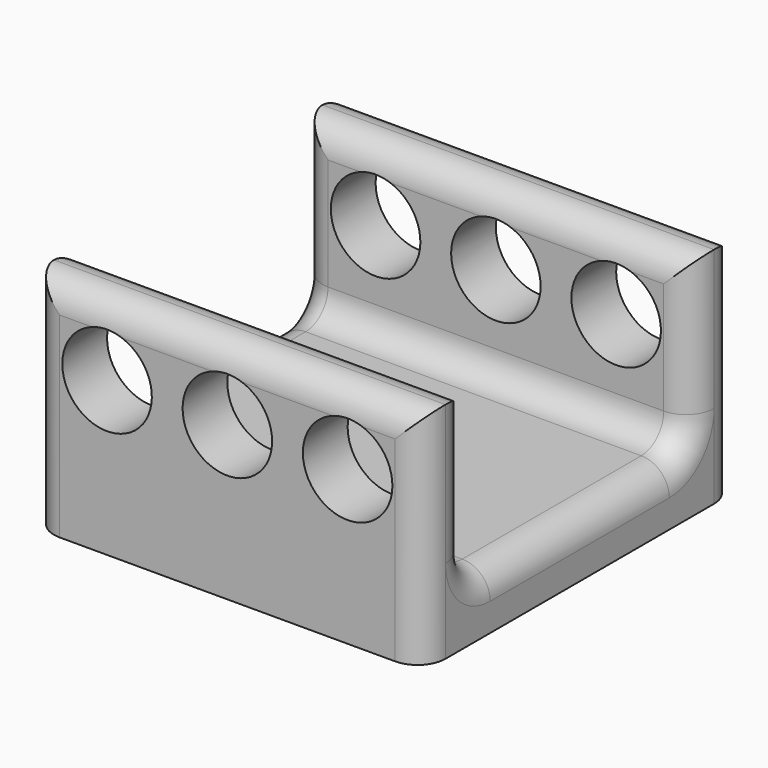
from build123d import *

# Parameters (mm, degrees)
F0_W         = 70
F0_H         = 70
F1_DEPTH     = 40
F3_DEPTH     = 78
F4_W         = 25
F4_H         = 17.3788098246
F5_DEPTH     = 72.2
F6_T1_DEPTH  = 70
F6_T3_DEPTH  = 40
F6_T5_DEPTH  = 65
F6_T7_DEPTH  = 37.5
F6_T9_DEPTH  = 95
F6_T12_ANGLE = 90
F6_T14_ANGLE = 90
F6_T16_ANGLE = 90
F6_T18_ANGLE = 90


# Not quite as in the source:
# - a fillet or chamfer that OpenCascade refuses, or shapes differently, is made with other operations: its cross-section is extruded or revolved along the edge and cut away or added
# - a feature names something its author has since deleted; it is built from what else it names


with BuildPart() as f1:
    # F0 (on Top) → F1 (new body)
    with BuildSketch(Plane.XY):
        Rectangle(F0_W, F0_H)
    extrude(amount=F1_DEPTH)

    # F2 (on face) → F3 (cut)
    with BuildSketch(Plane.XZ.offset(35)):
        with BuildLine():
            ThreePointArc((29.5, 27.4665858597), (21.5, 35.4665858597), (13.5, 27.4665858597))
            ThreePointArc((13.5, 27.4665858597), (21.5, 19.4665858597), (29.5, 27.4665858597))
        make_face()
        with BuildLine():
            ThreePointArc((8, 27.4665858597), (0, 35.4665858597), (-8, 27.4665858597))
            ThreePointArc((-8, 27.4665858597), (0, 19.4665858597), (8, 27.4665858597))
        make_face()
        with BuildLine():
            ThreePointArc((-13.5, 27.4665858597), (-21.5, 35.4665858597), (-29.5, 27.4665858597))
            ThreePointArc((-29.5, 27.4665858597), (-21.5, 19.4665858597), (-13.5, 27.4665858597))
        make_face()
    extrude(amount=-F3_DEPTH, mode=Mode.SUBTRACT)

    # F4 (on face) → F5 (cut)
    with BuildSketch(Plane(origin=(-35, 0, 0), x_dir=(0, -1, 0), z_dir=(-1, 0, 0))):
        with Locations((-12.5, 31.3105950877)):
            Rectangle(F4_W, F4_H)
        with Locations((12.5, 31.3105950877)):
            Rectangle(F4_W, F4_H)
        Polygon((25, 22.6211901754), (0, 22.6211901754), (-25, 22.6211901754), (-25, 10), (25, 10), align=None)
    extrude(amount=-F5_DEPTH, mode=Mode.SUBTRACT)

    # F6: fillet of radius 5 on 16 edges, made by hand

    # F6_s2 → F6_t1 (join)
    with BuildSketch(Plane.YZ.offset(-35)):
        with BuildLine():
            ThreePointArc((20, 10), (23.5355339059, 11.4644660941), (25, 15))
            Line((25, 15), (25, 10))
            Line((25, 10), (20, 10))
        make_face()
        with BuildLine():
            ThreePointArc((-25, 15), (-23.5355339059, 11.4644660941), (-20, 10))
            Line((-20, 10), (-25, 10))
            Line((-25, 10), (-25, 15))
        make_face()
    extrude(amount=F6_T1_DEPTH)

    # F6_s4 → F6_t3 (cut)
    with BuildSketch(Plane.XZ.offset(-20)):
        with BuildLine():
            ThreePointArc((35, 5), (33.5355339059, 8.5355339059), (30, 10))
            Line((30, 10), (35, 10))
            Line((35, 10), (35, 5))
        make_face()
        with BuildLine():
            ThreePointArc((-35, 5), (-33.5355339059, 8.5355339059), (-30, 10))
            Line((-30, 10), (-35, 10))
            Line((-35, 10), (-35, 5))
        make_face()
    extrude(amount=F6_T3_DEPTH, mode=Mode.SUBTRACT)

    # F6_s6 → F6_t5 (cut)
    with BuildSketch(Plane.XY.offset(-12.5)):
        with BuildLine():
            ThreePointArc((30, -35), (33.5355339059, -33.5355339059), (35, -30))
            Line((35, -30), (35, -35))
            Line((35, -35), (30, -35))
        make_face()
        with BuildLine():
            ThreePointArc((35, 30), (33.5355339059, 33.5355339059), (30, 35))
            Line((30, 35), (35, 35))
            Line((35, 35), (35, 30))
        make_face()
        with BuildLine():
            ThreePointArc((-35, 30), (-33.5355339059, 33.5355339059), (-30, 35))
            Line((-30, 35), (-35, 35))
            Line((-35, 35), (-35, 30))
        make_face()
        with BuildLine():
            ThreePointArc((-30, -35), (-33.5355339059, -33.5355339059), (-35, -30))
            Line((-35, -30), (-35, -35))
            Line((-35, -35), (-30, -35))
        make_face()
    extrude(amount=F6_T5_DEPTH, mode=Mode.SUBTRACT)

    # F6_s8 → F6_t7 (cut)
    with BuildSketch(Plane.XY.offset(15)):
        with BuildLine():
            ThreePointArc((-35, 30), (-33.5355339059, 26.4644660941), (-30, 25))
            Line((-30, 25), (-35, 25))
            Line((-35, 25), (-35, 30))
        make_face()
        with BuildLine():
            ThreePointArc((-35, -30), (-33.5355339059, -26.4644660941), (-30, -25))
            Line((-30, -25), (-35, -25))
            Line((-35, -25), (-35, -30))
        make_face()
        with BuildLine():
            ThreePointArc((35, 30), (33.5355339059, 26.4644660941), (30, 25))
            Line((30, 25), (35, 25))
            Line((35, 25), (35, 30))
        make_face()
        with BuildLine():
            ThreePointArc((35, -30), (33.5355339059, -26.4644660941), (30, -25))
            Line((30, -25), (35, -25))
            Line((35, -25), (35, -30))
        make_face()
    extrude(amount=F6_T7_DEPTH, mode=Mode.SUBTRACT)

    # F6_s10 → F6_t9 (cut)
    with BuildSketch(Plane.YZ.offset(-47.5)):
        with BuildLine():
            ThreePointArc((-30, 40), (-26.4644660941, 38.5355339059), (-25, 35))
            Line((-25, 35), (-25, 40))
            Line((-25, 40), (-30, 40))
        make_face()
        with BuildLine():
            ThreePointArc((-35, 35), (-33.5355339059, 38.5355339059), (-30, 40))
            Line((-30, 40), (-35, 40))
            Line((-35, 40), (-35, 35))
        make_face()
        with BuildLine():
            ThreePointArc((30, 40), (33.5355339059, 38.5355339059), (35, 35))
            Line((35, 35), (35, 40))
            Line((35, 40), (30, 40))
        make_face()
        with BuildLine():
            ThreePointArc((25, 35), (26.4644660941, 38.5355339059), (30, 40))
            Line((30, 40), (25, 40))
            Line((25, 40), (25, 35))
        make_face()
    extrude(amount=F6_T9_DEPTH, mode=Mode.SUBTRACT)

    # F6_s11 → F6_t12 (revolve, cut)
    with BuildSketch(Plane.XY.offset(15)):
        with BuildLine():
            ThreePointArc((35, -30), (33.5355339059, -26.4644660941), (30, -25))
            Line((30, -25), (35, -25))
            Line((35, -25), (35, -30))
        make_face()
    revolve(axis=Axis((35, -20, 15), (1, 0, 0)), revolution_arc=F6_T12_ANGLE, mode=Mode.SUBTRACT)

    # F6_s13 → F6_t14 (revolve, cut)
    with BuildSketch(Plane.XZ.offset(-20)):
        with BuildLine():
            ThreePointArc((35, 5), (33.5355339059, 8.5355339059), (30, 10))
            Line((30, 10), (35, 10))
            Line((35, 10), (35, 5))
        make_face()
    revolve(axis=Axis((35, 20, 15), (1, 0, 0)), revolution_arc=F6_T14_ANGLE, mode=Mode.SUBTRACT)

    # F6_s15 → F6_t16 (revolve, cut)
    with BuildSketch(Plane.XZ.offset(-20)):
        with BuildLine():
            ThreePointArc((-35, 5), (-33.5355339059, 8.5355339059), (-30, 10))
            Line((-30, 10), (-35, 10))
            Line((-35, 10), (-35, 5))
        make_face()
    revolve(axis=Axis((-35, 20, 15), (1, 0, 0)), revolution_arc=F6_T16_ANGLE, mode=Mode.SUBTRACT)

    # F6_s17 → F6_t18 (revolve, cut)
    with BuildSketch(Plane.XY.offset(15)):
        with BuildLine():
            ThreePointArc((-35, -30), (-33.5355339059, -26.4644660941), (-30, -25))
            Line((-30, -25), (-35, -25))
            Line((-35, -25), (-35, -30))
        make_face()
    revolve(axis=Axis((-35, -20, 15), (1, 0, 0)), revolution_arc=F6_T18_ANGLE, mode=Mode.SUBTRACT)


solid = f1.part
